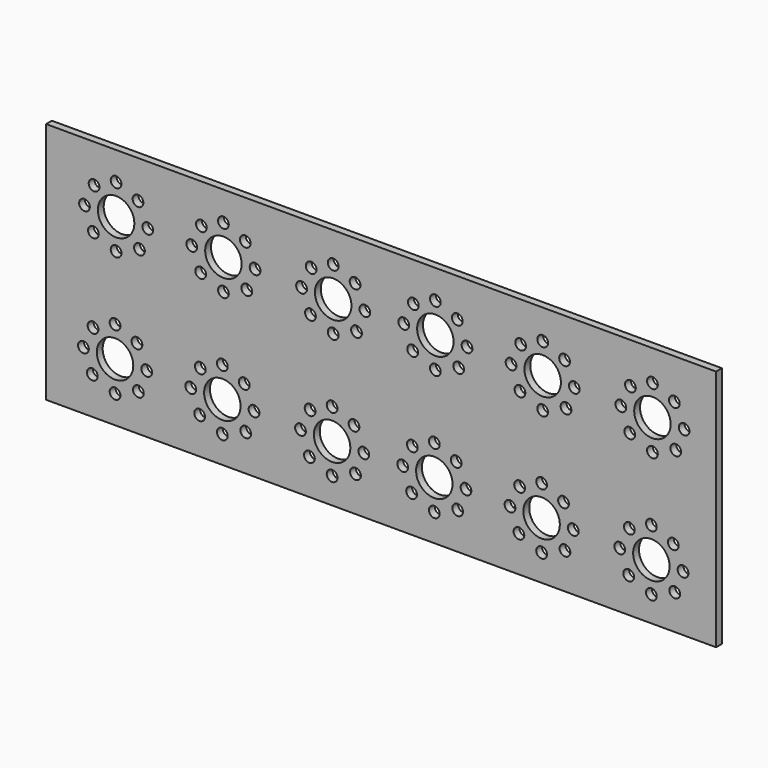
from build123d import *

# Parameters (mm, degrees)
F0_W     = 233.4336936474
F0_H     = 84.5690276474
F0_R     = 1.8721957215
F0_R_2   = 6.35
F1_DEPTH = 2.54


# Not quite as in the source:
# - a feature names something its author has since deleted; it is built from what else it names


with BuildPart() as f1:
    # F0 (on Front) → F1 (new body)
    with BuildSketch(Plane.XZ):
        with Locations((-11.6664916277, 61.8299962953)):
            Rectangle(F0_W, F0_H)
        with Locations((-104.3571985153, 29.2857964082)):
            Circle(F0_R, mode=Mode.SUBTRACT)
        with Locations((-112.2689694166, 32.5818173587)):
            Circle(F0_R, mode=Mode.SUBTRACT)
        with Locations((-115.3711608437, 39.9046507223)):
            Circle(F0_R, mode=Mode.SUBTRACT)
        with Locations((-104.3571985153, 39.9046507223)):
            Circle(F0_R_2, mode=Mode.SUBTRACT)
        with Locations((-96.2211242398, 32.574690507)):
            Circle(F0_R, mode=Mode.SUBTRACT)
        with Locations((-74.883861413, 32.3070631458)):
            Circle(F0_R, mode=Mode.SUBTRACT)
        with Locations((-93.3202734975, 39.9046507223)):
            Circle(F0_R, mode=Mode.SUBTRACT)
        with Locations((-77.9860528401, 39.6298965093)):
            Circle(F0_R, mode=Mode.SUBTRACT)
        with Locations((-66.9720905117, 29.0110421952)):
            Circle(F0_R, mode=Mode.SUBTRACT)
        with Locations((-28.7286259285, 28.620999728)):
            Circle(F0_R, mode=Mode.SUBTRACT)
        with Locations((-58.8360162362, 32.299936294)):
            Circle(F0_R, mode=Mode.SUBTRACT)
        with Locations((-66.9720905117, 39.6298965093)):
            Circle(F0_R_2, mode=Mode.SUBTRACT)
        with Locations((-55.9351654939, 39.6298965093)):
            Circle(F0_R, mode=Mode.SUBTRACT)
        with Locations((-36.6403968299, 31.9170206785)):
            Circle(F0_R, mode=Mode.SUBTRACT)
        with Locations((-20.5925516531, 31.9098938268)):
            Circle(F0_R, mode=Mode.SUBTRACT)
        with Locations((-39.742588257, 39.2398540421)):
            Circle(F0_R, mode=Mode.SUBTRACT)
        with Locations((-28.7286259285, 39.2398540421)):
            Circle(F0_R_2, mode=Mode.SUBTRACT)
        with Locations((-17.6917009107, 39.2398540421)):
            Circle(F0_R, mode=Mode.SUBTRACT)
        with Locations((-112.0281557075, 47.0351953909)):
            Circle(F0_R, mode=Mode.SUBTRACT)
        with Locations((-104.3571985153, 50.5235087617)):
            Circle(F0_R, mode=Mode.SUBTRACT)
        with Locations((-96.7241733432, 47.2419499663)):
            Circle(F0_R, mode=Mode.SUBTRACT)
        with Locations((-74.6430477039, 46.7604411779)):
            Circle(F0_R, mode=Mode.SUBTRACT)
        with Locations((-59.3390653396, 46.9671957533)):
            Circle(F0_R, mode=Mode.SUBTRACT)
        with Locations((-66.9720905117, 50.2487545487)):
            Circle(F0_R, mode=Mode.SUBTRACT)
        with Locations((-36.3995831207, 46.3703987107)):
            Circle(F0_R, mode=Mode.SUBTRACT)
        with Locations((-28.7286259285, 49.8587120814)):
            Circle(F0_R, mode=Mode.SUBTRACT)
        with Locations((-21.0956007565, 46.5771532861)):
            Circle(F0_R, mode=Mode.SUBTRACT)
        with Locations((6.8762816883, 29.1194615197)):
            Circle(F0_R, mode=Mode.SUBTRACT)
        with Locations((44.2613896919, 28.8447073068)):
            Circle(F0_R, mode=Mode.SUBTRACT)
        with Locations((-1.035489213, 32.4154824703)):
            Circle(F0_R, mode=Mode.SUBTRACT)
        with Locations((15.0123559638, 32.4083556185)):
            Circle(F0_R, mode=Mode.SUBTRACT)
        with Locations((-4.1376806401, 39.7383158338)):
            Circle(F0_R, mode=Mode.SUBTRACT)
        with Locations((6.8762816883, 39.7383158338)):
            Circle(F0_R_2, mode=Mode.SUBTRACT)
        with Locations((36.3496187906, 32.1407282573)):
            Circle(F0_R, mode=Mode.SUBTRACT)
        with Locations((17.9132067062, 39.7383158338)):
            Circle(F0_R, mode=Mode.SUBTRACT)
        with Locations((33.2474273635, 39.4635616208)):
            Circle(F0_R, mode=Mode.SUBTRACT)
        with Locations((44.2613896919, 39.4635616208)):
            Circle(F0_R_2, mode=Mode.SUBTRACT)
        with Locations((82.5048542751, 28.4546648395)):
            Circle(F0_R, mode=Mode.SUBTRACT)
        with Locations((52.3974639674, 32.1336014056)):
            Circle(F0_R, mode=Mode.SUBTRACT)
        with Locations((74.5930833738, 31.7506857901)):
            Circle(F0_R, mode=Mode.SUBTRACT)
        with Locations((55.2983147098, 39.4635616208)):
            Circle(F0_R, mode=Mode.SUBTRACT)
        with Locations((71.4908919467, 39.0735191536)):
            Circle(F0_R, mode=Mode.SUBTRACT)
        with Locations((90.6409285506, 31.7435589383)):
            Circle(F0_R, mode=Mode.SUBTRACT)
        with Locations((82.5048542751, 39.0735191536)):
            Circle(F0_R_2, mode=Mode.SUBTRACT)
        with Locations((93.5417792929, 39.0735191536)):
            Circle(F0_R, mode=Mode.SUBTRACT)
        with Locations((-0.7946755039, 46.8688605024)):
            Circle(F0_R, mode=Mode.SUBTRACT)
        with Locations((14.5093068604, 47.0756150778)):
            Circle(F0_R, mode=Mode.SUBTRACT)
        with Locations((6.8762816883, 50.3571738732)):
            Circle(F0_R, mode=Mode.SUBTRACT)
        with Locations((36.5904324997, 46.5941062895)):
            Circle(F0_R, mode=Mode.SUBTRACT)
        with Locations((44.2613896919, 50.0824196602)):
            Circle(F0_R, mode=Mode.SUBTRACT)
        with Locations((51.894414864, 46.8008608649)):
            Circle(F0_R, mode=Mode.SUBTRACT)
        with Locations((74.8338970829, 46.2040638222)):
            Circle(F0_R, mode=Mode.SUBTRACT)
        with Locations((90.1378794472, 46.4108183976)):
            Circle(F0_R, mode=Mode.SUBTRACT)
        with Locations((82.5048542751, 49.692377193)):
            Circle(F0_R, mode=Mode.SUBTRACT)
        with Locations((-103.9882795885, 73.0159394443)):
            Circle(F0_R, mode=Mode.SUBTRACT)
        with Locations((-111.9000504898, 76.3119603949)):
            Circle(F0_R, mode=Mode.SUBTRACT)
        with Locations((-95.852205313, 76.3048335431)):
            Circle(F0_R, mode=Mode.SUBTRACT)
        with Locations((-74.5149424862, 76.0372061819)):
            Circle(F0_R, mode=Mode.SUBTRACT)
        with Locations((-28.3597070018, 72.3511427641)):
            Circle(F0_R, mode=Mode.SUBTRACT)
        with Locations((-66.6031715849, 72.7411852313)):
            Circle(F0_R, mode=Mode.SUBTRACT)
        with Locations((-58.4670973094, 76.0300793301)):
            Circle(F0_R, mode=Mode.SUBTRACT)
        with Locations((-36.2714779031, 75.6471637146)):
            Circle(F0_R, mode=Mode.SUBTRACT)
        with Locations((-20.2236327263, 75.6400368629)):
            Circle(F0_R, mode=Mode.SUBTRACT)
        with Locations((-39.3736693302, 82.9699970782)):
            Circle(F0_R, mode=Mode.SUBTRACT)
        with Locations((-28.3597070018, 82.9699970782)):
            Circle(F0_R_2, mode=Mode.SUBTRACT)
        with Locations((-17.3227819839, 82.9699970782)):
            Circle(F0_R, mode=Mode.SUBTRACT)
        with Locations((-115.002241917, 83.6347937584)):
            Circle(F0_R, mode=Mode.SUBTRACT)
        with Locations((-103.9882795885, 83.6347937584)):
            Circle(F0_R_2, mode=Mode.SUBTRACT)
        with Locations((-111.6592367807, 90.765338427)):
            Circle(F0_R, mode=Mode.SUBTRACT)
        with Locations((-92.9513545707, 83.6347937584)):
            Circle(F0_R, mode=Mode.SUBTRACT)
        with Locations((-77.6171339134, 83.3600395454)):
            Circle(F0_R, mode=Mode.SUBTRACT)
        with Locations((-96.3552544164, 90.9720930024)):
            Circle(F0_R, mode=Mode.SUBTRACT)
        with Locations((-74.2741287771, 90.490584214)):
            Circle(F0_R, mode=Mode.SUBTRACT)
        with Locations((-103.9882795885, 94.2536517978)):
            Circle(F0_R, mode=Mode.SUBTRACT)
        with Locations((-66.6031715849, 83.3600395454)):
            Circle(F0_R_2, mode=Mode.SUBTRACT)
        with Locations((-55.5662465671, 83.3600395454)):
            Circle(F0_R, mode=Mode.SUBTRACT)
        with Locations((-58.9701464129, 90.6973387894)):
            Circle(F0_R, mode=Mode.SUBTRACT)
        with Locations((-36.030664194, 90.1005417468)):
            Circle(F0_R, mode=Mode.SUBTRACT)
        with Locations((-20.7266818297, 90.3072963222)):
            Circle(F0_R, mode=Mode.SUBTRACT)
        with Locations((-66.6031715849, 93.9788975848)):
            Circle(F0_R, mode=Mode.SUBTRACT)
        with Locations((-28.3597070018, 93.5888551176)):
            Circle(F0_R, mode=Mode.SUBTRACT)
        with Locations((-0.6665702862, 76.1456255064)):
            Circle(F0_R, mode=Mode.SUBTRACT)
        with Locations((7.2452006151, 72.8496045558)):
            Circle(F0_R, mode=Mode.SUBTRACT)
        with Locations((15.3812748906, 76.1384986547)):
            Circle(F0_R, mode=Mode.SUBTRACT)
        with Locations((44.6303086187, 72.5748503429)):
            Circle(F0_R, mode=Mode.SUBTRACT)
        with Locations((36.7185377174, 75.8708712934)):
            Circle(F0_R, mode=Mode.SUBTRACT)
        with Locations((82.8737732019, 72.1848078756)):
            Circle(F0_R, mode=Mode.SUBTRACT)
        with Locations((52.7663828942, 75.8637444417)):
            Circle(F0_R, mode=Mode.SUBTRACT)
        with Locations((74.9620023005, 75.4808288262)):
            Circle(F0_R, mode=Mode.SUBTRACT)
        with Locations((71.8598108734, 82.8036621897)):
            Circle(F0_R, mode=Mode.SUBTRACT)
        with Locations((91.0098474773, 75.4737019744)):
            Circle(F0_R, mode=Mode.SUBTRACT)
        with Locations((82.8737732019, 82.8036621897)):
            Circle(F0_R_2, mode=Mode.SUBTRACT)
        with Locations((93.9106982197, 82.8036621897)):
            Circle(F0_R, mode=Mode.SUBTRACT)
        with Locations((-3.7687617133, 83.4684588699)):
            Circle(F0_R, mode=Mode.SUBTRACT)
        with Locations((7.2452006151, 83.4684588699)):
            Circle(F0_R_2, mode=Mode.SUBTRACT)
        with Locations((-0.4257565771, 90.5990035386)):
            Circle(F0_R, mode=Mode.SUBTRACT)
        with Locations((14.8782257872, 90.805758114)):
            Circle(F0_R, mode=Mode.SUBTRACT)
        with Locations((18.2821256329, 83.4684588699)):
            Circle(F0_R, mode=Mode.SUBTRACT)
        with Locations((33.6163462903, 83.193704657)):
            Circle(F0_R, mode=Mode.SUBTRACT)
        with Locations((44.6303086187, 83.193704657)):
            Circle(F0_R_2, mode=Mode.SUBTRACT)
        with Locations((36.9593514265, 90.3242493256)):
            Circle(F0_R, mode=Mode.SUBTRACT)
        with Locations((7.2452006151, 94.0873169093)):
            Circle(F0_R, mode=Mode.SUBTRACT)
        with Locations((44.6303086187, 93.8125626963)):
            Circle(F0_R, mode=Mode.SUBTRACT)
        with Locations((55.6672336365, 83.193704657)):
            Circle(F0_R, mode=Mode.SUBTRACT)
        with Locations((52.2633337908, 90.531003901)):
            Circle(F0_R, mode=Mode.SUBTRACT)
        with Locations((75.2028160097, 89.9342068583)):
            Circle(F0_R, mode=Mode.SUBTRACT)
        with Locations((82.8737732019, 93.4225202291)):
            Circle(F0_R, mode=Mode.SUBTRACT)
        with Locations((90.5067983739, 90.1409614337)):
            Circle(F0_R, mode=Mode.SUBTRACT)
    extrude(amount=F1_DEPTH)


solid = f1.part
